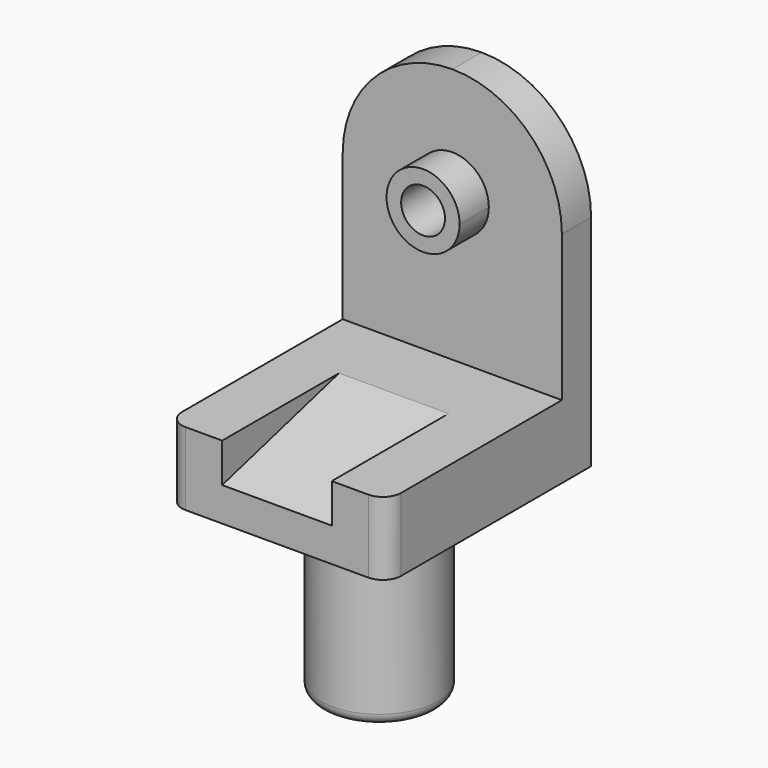
from build123d import *

# Parameters (mm, degrees)
F0_R      = 16
F1_DEPTH  = 50
F4_R      = 3
F5_W      = 30
F5_H      = 40
F6_DEPTH  = 20
F8_DEPTH  = 15
F9_DEPTH  = 20
F11_W     = 60
F11_H     = 10
F12_DEPTH = 70
F13_R     = 29.99999
F16_DEPTH = 10
F18_R     = 6
F19_DEPTH = 50
F20_R     = 5


# Not quite as in the source:
# - a fillet or chamfer is up to 0.001 mm smaller than in the source, because OpenCascade refuses the exact size


with BuildPart() as f1:
    # F0 (on Top) → F1 (new body)
    with BuildSketch(Plane.XY):
        Circle(F0_R)
    extrude(amount=F1_DEPTH)

    # F4
    f4_edges = [f1.edges().sort_by_distance(p)[0] for p in [
        (-16, 0, 0),
    ]]
    fillet(f4_edges, radius=F4_R)

    # F5 (on offset) → F6 (join)
    with BuildSketch(Plane.XY.offset(50)):
        with Locations((0, -15)):
            Rectangle(F5_W, F5_H)
    extrude(amount=F6_DEPTH)

    # F7 (on Right) → F8 (cut, symmetric)
    with BuildSketch(Plane.YZ):
        Polygon((5, 70), (0, 70), (-35, 70), (-35, 59.2820323028), align=None)
    extrude(amount=F8_DEPTH, both=True, mode=Mode.SUBTRACT)

    # F3 (on offset) → F9 (join)
    with BuildSketch(Plane.XY.offset(50)):
        Polygon((30, 35), (-30, 35), (-30, -35), (-15, -35), (-15, 5), (15, 5), (15, -35), (30, -35), align=None)
    extrude(amount=F9_DEPTH)

    # F11 (on offset) → F12 (join)
    with BuildSketch(Plane.XY.offset(70)):
        with Locations((0, 30)):
            Rectangle(F11_W, F11_H)
    extrude(amount=F12_DEPTH)

    # F13 (radius 30 in the source; OpenCascade refuses exactly that, so slightly less here)
    f13_edges = [f1.edges().sort_by_distance(p)[0] for p in [
        (-30, 30, 140),
        (30, 30, 140),
    ]]
    fillet(f13_edges, radius=F13_R)

    # F15 (on offset) → F16 (join)
    with BuildSketch(Plane.XZ.offset(-25)):
        with BuildLine():
            ThreePointArc((0, 100), (7.0710678119, 102.9289321881), (10, 110))
            ThreePointArc((10, 110), (-7.0710678119, 117.0710678119), (0, 100))
        make_face()
    extrude(amount=F16_DEPTH)

    # F18 (on offset) → F19 (cut)
    with BuildSketch(Plane.XZ.offset(-15)):
        with Locations((0, 110)):
            Circle(F18_R)
    extrude(amount=-F19_DEPTH, mode=Mode.SUBTRACT)

    # F20
    f20_edges = [f1.edges().sort_by_distance(p)[0] for p in [
        (-30, -35, 60),
        (30, -35, 60),
    ]]
    fillet(f20_edges, radius=F20_R)


solid = f1.part
